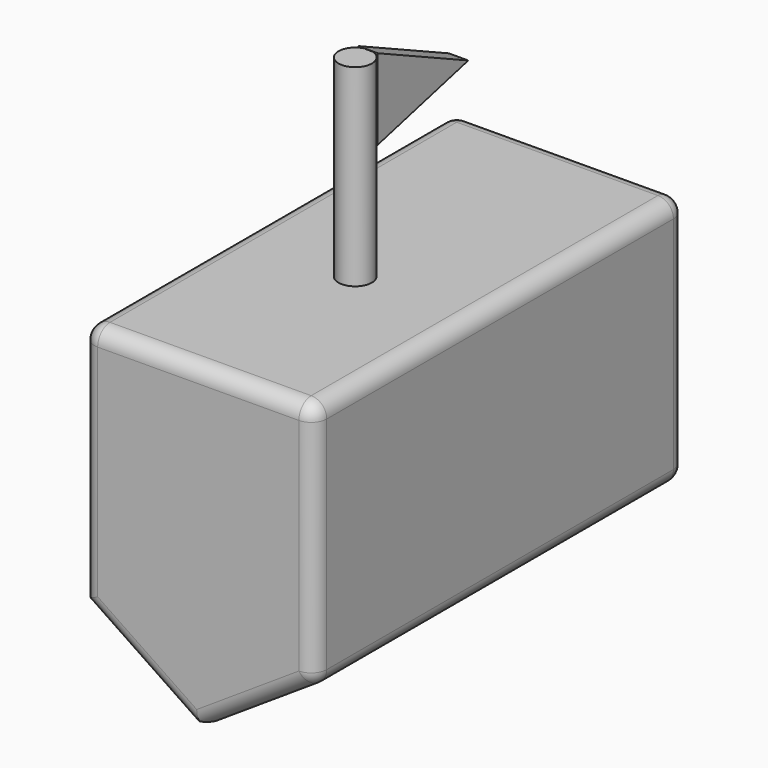
from build123d import *

# Parameters (mm, degrees)
F1_DEPTH     = 152.4
F2_T1_DEPTH  = 159.9639298233
F2_T3_DEPTH  = 87.5512753886
F2_T5_DEPTH  = 105.6460143168
F2_T7_DEPTH  = 83.8431740092
F2_T9_DEPTH  = 66.9209927252
F2_T11_DEPTH = 67.7625979145
F2_T16_DEPTH = 5.08
F4_W         = 5.4661177176
F4_H         = 63.5
F7_DEPTH     = 3.175
F8_T1_DEPTH  = 142.24
F8_T3_DEPTH  = 87.5512753886
F8_T5_DEPTH  = 66.9209927252
F8_T7_DEPTH  = 52.3221869503
F8_T9_DEPTH  = 72.4030758235
F8_T11_DEPTH = 66.0406464801
F8_T16_DEPTH = 5.08
F8_T22_DEPTH = 5.08
F8_T28_DEPTH = 5.08
F8_T34_DEPTH = 5.08
F8_T38_ANGLE = 89.746481368


# Not quite as in the source:
# - a fillet or chamfer that OpenCascade refuses, or shapes differently, is made with other operations: its cross-section is extruded or revolved along the edge and cut away or added


with BuildPart() as f1:
    # F0 (on Front) → F1 (new body)
    with BuildSketch(Plane.XZ):
        Polygon((17.4287217617, 50.174562376), (-58.7712782383, 49.8373953771), (-58.7712782383, -30.0714519408), (-24.3801281386, -53.3360523395), (-17.9739344996, -53.3360523395), (17.4287217617, -30.0714519408), align=None)
    extrude(amount=F1_DEPTH)

    # F2: fillet of radius 5.08 on 6 edges, made by hand

    # F2_s2 → F2_t1 (cut)
    with BuildSketch(Plane.XZ.offset(-12.6439298233)):
        with BuildLine():
            ThreePointArc((-53.7137558182, 49.859773719), (-57.2913189399, 48.3639700613), (-58.7712782383, 44.7798234478))
            Line((-58.7712782383, 44.7798234478), (-58.7712782383, 49.8373953771))
            Line((-58.7712782383, 49.8373953771), (-53.7137558182, 49.859773719))
        make_face()
    extrude(amount=F2_T1_DEPTH, mode=Mode.SUBTRACT)

    # F2_s4 → F2_t3 (cut)
    with BuildSketch(Plane.XY.offset(-42.7714519408)):
        with BuildLine():
            ThreePointArc((-58.7712782383, -147.32), (-57.2833806867, -150.9121024484), (-53.6912782383, -152.4))
            Line((-53.6912782383, -152.4), (-58.7712782383, -152.4))
            Line((-58.7712782383, -152.4), (-58.7712782383, -147.32))
        make_face()
    extrude(amount=F2_T3_DEPTH, mode=Mode.SUBTRACT)

    # F2_s6 → F2_t5 (cut)
    with BuildSketch(Plane.XY.offset(-42.7714519408)):
        with BuildLine():
            ThreePointArc((17.4287217617, -147.32), (15.9408242101, -150.9121024484), (12.3487217617, -152.4))
            Line((12.3487217617, -152.4), (17.4287217617, -152.4))
            Line((17.4287217617, -152.4), (17.4287217617, -147.32))
        make_face()
    extrude(amount=F2_T5_DEPTH, mode=Mode.SUBTRACT)

    # F2_s8 → F2_t7 (cut)
    with BuildSketch(Plane(origin=(30.3502624567, 0, 0.1342927416), x_dir=(0, 1, 0), z_dir=(-0.9999902109, 0, -0.0044247205))):
        with BuildLine():
            ThreePointArc((-147.32, -50.0969539894), (-150.9121024484, -48.6090564378), (-152.4, -45.0169539894))
            Line((-152.4, -45.0169539894), (-152.4, -50.0969539894))
            Line((-152.4, -50.0969539894), (-147.32, -50.0969539894))
        make_face()
    extrude(amount=F2_T7_DEPTH, mode=Mode.SUBTRACT)

    # F2_s10 → F2_t9 (cut)
    with BuildSketch(Plane(origin=(-36.8834278428, 0, 24.9505529071), x_dir=(0, 1, 0), z_dir=(0.8282834259, 0, -0.5603093489))):
        with BuildLine():
            ThreePointArc((-147.32, -57.8377818767), (-150.9121024484, -56.3498843251), (-152.4, -52.7577818767))
            Line((-152.4, -52.7577818767), (-152.4, -57.8377818767))
            Line((-152.4, -57.8377818767), (-147.32, -57.8377818767))
        make_face()
    extrude(amount=F2_T9_DEPTH, mode=Mode.SUBTRACT)

    # F2_s12 → F2_t11 (cut)
    with BuildSketch(Plane(origin=(-47.6451540495, 0, -31.3096695828), x_dir=(0, 1, 0), z_dir=(0.8357055045, 0, 0.549177849))):
        with BuildLine():
            ThreePointArc((-147.32, -34.7023458418), (-150.9121024484, -33.2144482902), (-152.4, -29.6223458418))
            Line((-152.4, -29.6223458418), (-152.4, -34.7023458418))
            Line((-152.4, -34.7023458418), (-147.32, -34.7023458418))
        make_face()
    extrude(amount=F2_T11_DEPTH, mode=Mode.SUBTRACT)


with BuildPart() as f2_tool14:
    # F2_s15 → F2_t16 (new body)
    with BuildSketch(Plane.XZ.offset(147.32)):
        Polygon((-53.6912782383, 44.7798234478), (-53.7137558182, 49.859773719), (-58.7712782383, 49.8373953771), (-58.7712782383, 44.7798234478), align=None)
    extrude(amount=F2_T16_DEPTH)

    # F2_s17 → F2_t18 (revolve, cut)
    with BuildSketch(Plane(origin=(-53.6912782383, -147.32, 44.7798234478), x_dir=(0.7086694294, 0, -0.7055406719), z_dir=(-0.7055406719, 0, -0.7086694294))):
        with BuildLine():
            ThreePointArc((0, -5.08), (5.08, 0), (0, 5.08))
            Line((0, 5.08), (0, -5.08))
        make_face()
    revolve(axis=Axis((-53.6912782383, -147.32, 44.7798234478), (0, -1, 0)), mode=Mode.SUBTRACT)


with BuildPart() as f1_1:
    add(f1.part)

    # F2_t13: cut F2_tool14
    add(f2_tool14.part, mode=Mode.SUBTRACT)

    # F4 (on offset) → F5 (revolve)
    with BuildSketch(Plane.YZ.offset(-20.32)):
        with Locations((-85.7021328023, 81.609773719)):
            Rectangle(F4_W, F4_H)
    revolve(axis=Axis((-20.32, -88.4351916611, 88.4142501174), (0, 0, 1)))

    # F6 (on offset) → F7 (join, symmetric)
    with BuildSketch(Plane.YZ.offset(-20.32)):
        Polygon((-46.0359752178, 96.2450280786), (-83.1919163465, 113.4468540549), (-83.1919163465, 86.9560390711), align=None)
    extrude(amount=F7_DEPTH, both=True)

    # F8: fillet of radius 5.08 on 8 edges, made by hand

    # F8_s2 → F8_t1 (cut)
    with BuildSketch(Plane.XZ.offset(5.08)):
        with BuildLine():
            ThreePointArc((12.3262441818, 50.1519851181), (15.9328683752, 48.6720755484), (17.4287217617, 45.0720348468))
            Line((17.4287217617, 45.0720348468), (17.4287217617, 50.174562376))
            Line((17.4287217617, 50.174562376), (12.3262441818, 50.1519851181))
        make_face()
        with BuildLine():
            ThreePointArc((15.1385452344, -31.5764249394), (16.8196670332, -29.7428967724), (17.4287217617, -27.3310409766))
            Line((17.4287217617, -27.3310409766), (17.4287217617, -30.0714519408))
            Line((17.4287217617, -30.0714519408), (15.1385452344, -31.5764249394))
        make_face()
    extrude(amount=F8_T1_DEPTH, mode=Mode.SUBTRACT)

    # F8_s4 → F8_t3 (cut)
    with BuildSketch(Plane.XY.offset(-42.7714519408)):
        with BuildLine():
            ThreePointArc((-58.7712782383, -5.08), (-57.2833806867, -1.4878975516), (-53.6912782383, 0))
            Line((-53.6912782383, 0), (-58.7712782383, 0))
            Line((-58.7712782383, 0), (-58.7712782383, -5.08))
        make_face()
    extrude(amount=F8_T3_DEPTH, mode=Mode.SUBTRACT)

    # F8_s6 → F8_t5 (cut)
    with BuildSketch(Plane(origin=(-36.8834278428, 0, 24.9505529071), x_dir=(0, 1, 0), z_dir=(0.8282834259, 0, -0.5603093489))):
        with BuildLine():
            ThreePointArc((-5.08, -57.8377818767), (-1.4878975516, -56.3498843251), (0, -52.7577818767))
            Line((0, -52.7577818767), (0, -57.8377818767))
            Line((0, -57.8377818767), (-5.08, -57.8377818767))
        make_face()
    extrude(amount=F8_T5_DEPTH, mode=Mode.SUBTRACT)

    # F8_s8 → F8_t7 (cut)
    with BuildSketch(Plane(origin=(-47.6451540495, 0, -31.3096695828), x_dir=(0, 1, 0), z_dir=(0.8357055045, 0, 0.549177849))):
        with BuildLine():
            ThreePointArc((-5.08, -34.7023458418), (-1.4878975516, -33.2144482902), (0, -29.6223458418))
            Line((0, -29.6223458418), (0, -34.7023458418))
            Line((0, -34.7023458418), (-5.08, -34.7023458418))
        make_face()
    extrude(amount=F8_T7_DEPTH, mode=Mode.SUBTRACT)

    # F8_s10 → F8_t9 (cut)
    with BuildSketch(Plane.XY.offset(-27.3310409766)):
        with BuildLine():
            ThreePointArc((17.4287217617, -5.08), (15.9408242101, -1.4878975516), (12.3487217617, 0))
            Line((12.3487217617, 0), (17.4287217617, 0))
            Line((17.4287217617, 0), (17.4287217617, -5.08))
        make_face()
    extrude(amount=F8_T9_DEPTH, mode=Mode.SUBTRACT)

    # F8_s12 → F8_t11 (cut)
    with BuildSketch(Plane(origin=(12.5479091987, 0, 0.055521534), x_dir=(0, 1, 0), z_dir=(-0.9999902109, 0, -0.0044247205))):
        with BuildLine():
            ThreePointArc((-5.08, -50.0969539894), (-1.4878975516, -48.6090564378), (0, -45.0169539894))
            Line((0, -45.0169539894), (0, -50.0969539894))
            Line((0, -50.0969539894), (-5.08, -50.0969539894))
        make_face()
    extrude(amount=F8_T11_DEPTH, mode=Mode.SUBTRACT)


with BuildPart() as f8_tool14:
    # F8_s15 → F8_t16 (new body)
    with BuildSketch(Plane.XZ.offset(147.32)):
        Polygon((12.3487217617, -27.3310409766), (15.1385452344, -31.5764249394), (17.4287217617, -30.0714519408), (17.4287217617, -27.3310409766), align=None)
    extrude(amount=F8_T16_DEPTH)

    # F8_s17 → F8_t18 (revolve, cut)
    with BuildSketch(Plane(origin=(12.3487217617, -147.32, -27.3310409766), x_dir=(-0.8801073369, 0, 0.4747747629), z_dir=(0.4747747629, 0, 0.8801073369))):
        with BuildLine():
            ThreePointArc((0, -5.08), (5.08, 0), (0, 5.08))
            Line((0, 5.08), (0, -5.08))
        make_face()
    revolve(axis=Axis((12.3487217617, -147.32, -27.3310409766), (0, -1, 0)), mode=Mode.SUBTRACT)


with BuildPart() as f1_2:
    add(f1_1.part)

    # F8_t13: cut F8_tool14
    add(f8_tool14.part, mode=Mode.SUBTRACT)


with BuildPart() as f8_tool20:
    # F8_s21 → F8_t22 (new body)
    with BuildSketch(Plane.XZ.offset(147.32)):
        Polygon((12.3487217617, 45.0720348468), (12.3262441818, 50.1519851181), (17.4287217617, 50.174562376), (17.4287217617, 45.0720348468), align=None)
    extrude(amount=F8_T22_DEPTH)

    # F8_s23 → F8_t24 (revolve, cut)
    with BuildSketch(Plane(origin=(12.3487217617, -147.32, 45.0720348468), x_dir=(-0.7055406719, 0, -0.7086694294), z_dir=(-0.7086694294, 0, 0.7055406719))):
        with BuildLine():
            ThreePointArc((0, -5.08), (5.08, 0), (0, 5.08))
            Line((0, 5.08), (0, -5.08))
        make_face()
    revolve(axis=Axis((12.3487217617, -147.32, 45.0720348468), (0, -1, 0)), mode=Mode.SUBTRACT)


with BuildPart() as f1_3:
    add(f1_2.part)

    # F8_t19: cut F8_tool20
    add(f8_tool20.part, mode=Mode.SUBTRACT)


with BuildPart() as f8_tool26:
    # F8_s27 → F8_t28 (new body)
    with BuildSketch(Plane.XZ.offset(5.08)):
        Polygon((12.3487217617, 45.0720348468), (12.3262441818, 50.1519851181), (17.4287217617, 50.174562376), (17.4287217617, 45.0720348468), align=None)
    extrude(amount=-F8_T28_DEPTH)

    # F8_s29 → F8_t30 (revolve, cut)
    with BuildSketch(Plane(origin=(12.3487217617, -5.08, 45.0720348468), x_dir=(-0.7055406719, 0, -0.7086694294), z_dir=(0.7086694294, 0, -0.7055406719))):
        with BuildLine():
            ThreePointArc((0, -5.08), (5.08, 0), (0, 5.08))
            Line((0, 5.08), (0, -5.08))
        make_face()
    revolve(axis=Axis((12.3487217617, -5.08, 45.0720348468), (0, 1, 0)), mode=Mode.SUBTRACT)


with BuildPart() as f1_4:
    add(f1_3.part)

    # F8_t25: cut F8_tool26
    add(f8_tool26.part, mode=Mode.SUBTRACT)


with BuildPart() as f8_tool32:
    # F8_s33 → F8_t34 (new body)
    with BuildSketch(Plane.XZ.offset(5.08)):
        Polygon((12.3487217617, -27.3310409766), (15.1385452344, -31.5764249394), (17.4287217617, -30.0714519408), (17.4287217617, -27.3310409766), align=None)
    extrude(amount=-F8_T34_DEPTH)

    # F8_s35 → F8_t36 (revolve, cut)
    with BuildSketch(Plane(origin=(12.3487217617, -5.08, -27.3310409766), x_dir=(-0.8801073369, 0, 0.4747747629), z_dir=(-0.4747747629, 0, -0.8801073369))):
        with BuildLine():
            ThreePointArc((0, -5.08), (5.08, 0), (0, 5.08))
            Line((0, 5.08), (0, -5.08))
        make_face()
    revolve(axis=Axis((12.3487217617, -5.08, -27.3310409766), (0, 1, 0)), mode=Mode.SUBTRACT)


with BuildPart() as f1_5:
    add(f1_4.part)

    # F8_t31: cut F8_tool32
    add(f8_tool32.part, mode=Mode.SUBTRACT)

    # F8_s37 → F8_t38 (revolve, cut)
    with BuildSketch(Plane.XY.offset(44.7798234479)):
        with BuildLine():
            ThreePointArc((-58.7712782383, -5.08), (-57.2833806867, -1.4878975516), (-53.6912782383, 0))
            Line((-53.6912782383, 0), (-58.7712782383, 0))
            Line((-58.7712782383, 0), (-58.7712782383, -5.08))
        make_face()
    revolve(axis=Axis((-53.6912782384, 0, 44.7798234479), (0, 1, 0)), revolution_arc=F8_T38_ANGLE, mode=Mode.SUBTRACT)


solid = f1_5.part
